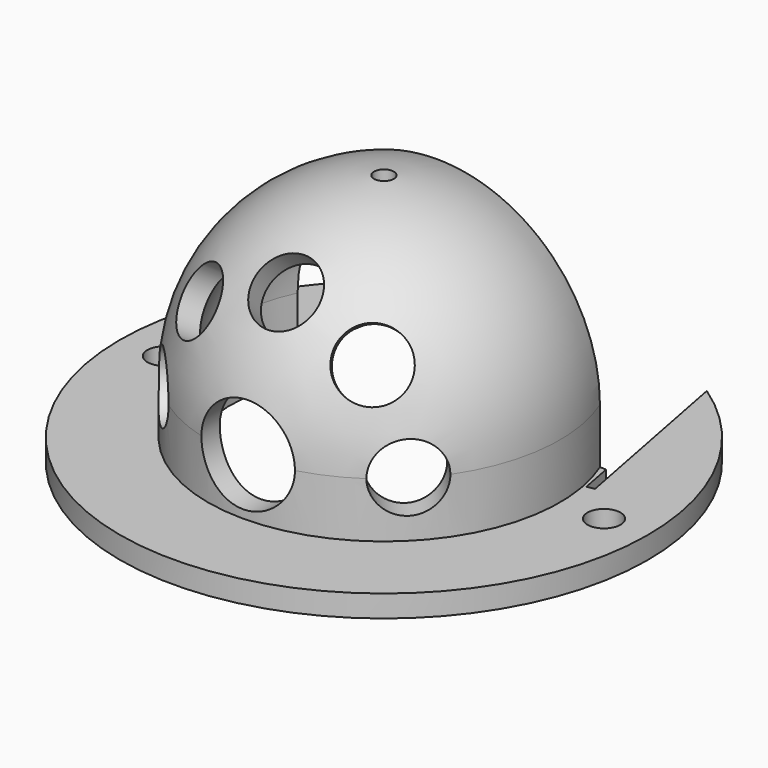
from build123d import *

# Parameters (mm, degrees)
F2_R             = 4.25
F3_DEPTH         = 50
F6_R             = 3
F7_DEPTH         = 25
F11_COPIES_COUNT = 3
F11_COPIES_ANGLE = 90
F13_R            = 3
F14_DEPTH        = 25
F17_R            = 0.9
F18_DEPTH        = 30.1
F24_DEPTH        = 29.9756674466
F25_R            = 1.5
F26_DEPTH        = 29.9756674466


# Not quite as in the source:
# - a pattern or mirror of a feature is missing from the dataset's text; its kind, count and spacing are read off the source's solid


with BuildPart() as f1:
    # F0 (on Front) → F1 (revolve)
    with BuildSketch(Plane.XZ):
        with BuildLine():
            Line((-24, -7), (-14, -7))
            Line((-14, -7), (-14, 0))
            ThreePointArc((-14, 0), (-9.8994949366, 9.8994949366), (0, 14))
            Line((0, 14), (0, 16))
            ThreePointArc((0, 16), (-11.313708499, 11.313708499), (-16, 0))
            Line((-16, 0), (-16, -5))
            Line((-16, -5), (-24, -5))
            Line((-24, -5), (-24, -7))
        make_face()
    revolve(axis=Axis((0, 0, 15), (0, 0, -1)))

    # F2 (on Front) → F3 (cut)
    with BuildSketch(Plane.XZ):
        Circle(F2_R)
    extrude(amount=F3_DEPTH, mode=Mode.SUBTRACT)

    # F6 (on face) → F7 (cut)
    with BuildSketch(Plane(origin=(0, 0, 0), x_dir=(-0.7071067812, 0.7071067812, 0), z_dir=(0.7071067812, 0.7071067812, 0))):
        Circle(F6_R)
    extrude(amount=-F7_DEPTH, mode=Mode.SUBTRACT)

    # F10 (on face) → F11 (revolve, cut)
    with BuildSketch(Plane(origin=(0, 0, 0), x_dir=(0, -1, 0), z_dir=(-0.7071067812, 0, 0.7071067812))):
        Polygon((3.9985278842, 3.9985278842), (16.6846810101, 16.6846810101), (14.5633606666, 18.8060013537), (1.8772075407, 6.1198482278), align=None)
    f11 = revolve(axis=Axis((7.3126186329, -10.3416044472, 7.3126186329), (0.5, -0.7071067812, 0.5)), mode=Mode.SUBTRACT)

    # F11_copies: F11 ×3 about axis
    f11_copies_axis = Axis((0, 0, 0), (0, -1, 0))
    for i in range(1, F11_COPIES_COUNT):
        add(f11.rotate(f11_copies_axis, i * F11_COPIES_ANGLE / (F11_COPIES_COUNT - 1)), mode=Mode.SUBTRACT)

    # F13 (on face) → F14 (cut)
    with BuildSketch(Plane(origin=(0, 0, 0), x_dir=(0.7071067812, 0.7071067812, 0), z_dir=(0.7071067812, -0.7071067812, 0))):
        Circle(F13_R)
    extrude(amount=F14_DEPTH, mode=Mode.SUBTRACT)

    # F17 (on Top) → F18 (cut)
    with BuildSketch(Plane.XY):
        Circle(F17_R)
    extrude(amount=F18_DEPTH, mode=Mode.SUBTRACT)

    # F23 (on offset) → F24 (cut, through all)
    with BuildSketch(Plane(origin=(0, 0, -14), x_dir=(1, 0, 0), z_dir=(0, 0, -1))):
        Polygon((15.39, -6), (-15.39, -6), (-15.956772168, -3.0540248966), (-16.6441663587, -3.1862717358), (-12.4878371271, -24.7900891605), (12.4878371271, -24.7900891605), (16.6441663587, -3.1862717358), (15.956772168, -3.0540248966), align=None)
    extrude(amount=-F24_DEPTH, mode=Mode.SUBTRACT)

    # F25 (on offset) → F26 (cut, through all)
    with BuildSketch(Plane(origin=(0, 0, -14), x_dir=(1, 0, 0), z_dir=(0, 0, -1))):
        with Locations((-20, 0)):
            Circle(F25_R)
        with Locations((20, 0)):
            Circle(F25_R)
    extrude(amount=-F26_DEPTH, mode=Mode.SUBTRACT)


solid = f1.part
